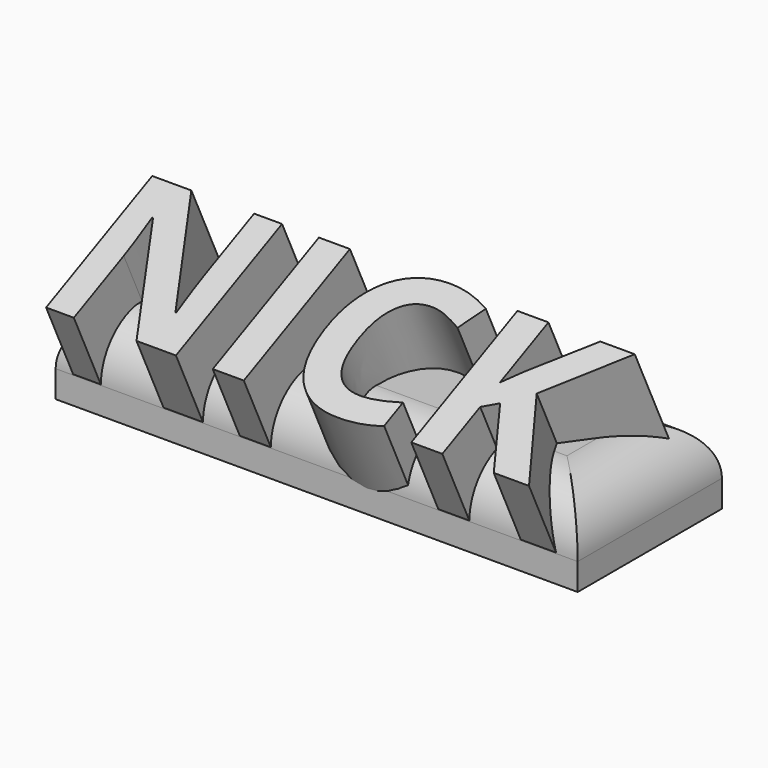
from build123d import *

# Parameters (mm, degrees)
F0_TEXT_SIZE = 38.1543249306
F1_DEPTH     = 20
F2_ANGLE     = -45
F3_W         = 97.1550010145
F3_H         = 33.5525814444
F4_DEPTH     = 15
F5_R         = 10
F7_ANGLE     = 20


# Not quite as in the source:
# - Text() gives the source's letters only with a copy of the font that has no kerning and outlines rounded to 1/6400 em; it was checked with that copy


with BuildPart() as f1:
    # F0 (on Top) → F1 (new body)
    with BuildSketch(Plane.XY):
        with Locations((-49.5725376531, -48.2163615525)):
            Text('NICK', F0_TEXT_SIZE, font='Open Sans', font_style=FontStyle.BOLD, text_align=(TextAlign.LEFT, TextAlign.BOTTOM))
    extrude(amount=F1_DEPTH)


with BuildPart() as f1_1:
    # F2: moved
    add(f1.part.rotate(Axis((-12.2379345473, -48.2163615525, 0), (-1, 0, 0)), F2_ANGLE))


with BuildPart() as f4:
    # F3 (on Top) → F4 (new body)
    with BuildSketch(Plane.XY):
        with Locations((4.5166928321, 4.2401617393)):
            Rectangle(F3_W, F3_H)
    extrude(amount=F4_DEPTH)

    # F5
    f5_edges = [f4.edges().sort_by_distance(p)[0] for p in [
        (-44.060808, 4.240162, 15),
        (4.516693, 21.016452, 15),
        (53.094193, 4.240162, 15),
        (4.516693, -12.536129, 15),
    ]]
    fillet(f5_edges, radius=F5_R)


with BuildPart() as f1_2:
    # F6: moved
    add(f1_1.part.moved(Location((5.334, 37.846, 0))))


with BuildPart() as f1_3:
    # F7: moved
    add(f1_2.part.rotate(Axis((-20.3175644057, -10.3703615525, 0), (-1, 0, 0)), F7_ANGLE))


with BuildPart() as f1_4:
    # F8: moved
    add(f1_3.part.moved(Location((0, 0, 0.508))))


solid = Compound([f4.part, f1_4.part])
